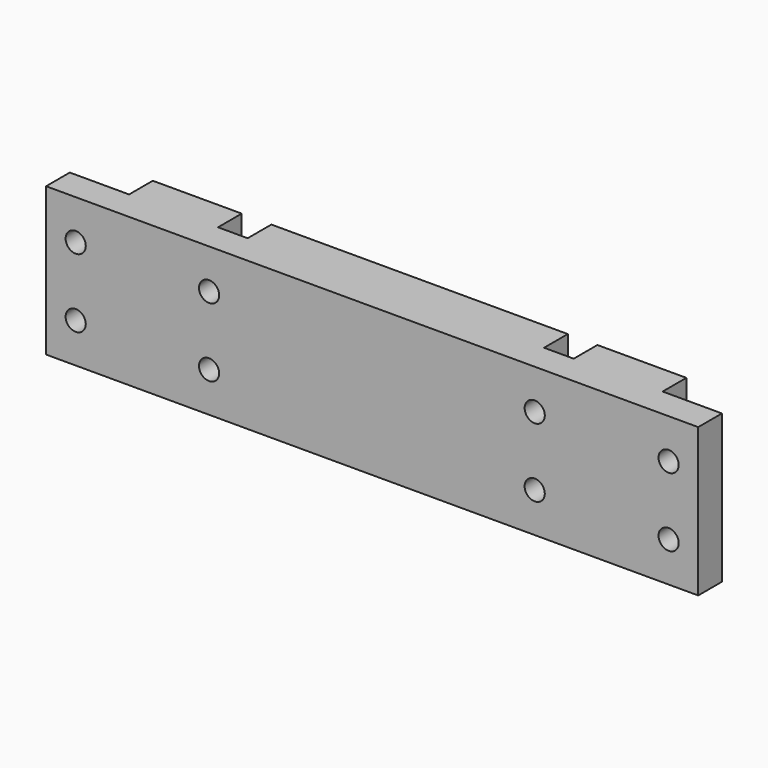
from build123d import *

# Parameters (mm, degrees)
F0_W      = 12.7
F0_H      = 31.75
F1_DEPTH  = 139.7
F2_W      = 12.7
F2_H      = 6.35
F2_W_2    = 6.35
F3_DEPTH  = 31.751
F4_R      = 2.159
F5_DEPTH  = 25.4
F6_R      = 2.159
F7_DEPTH  = 25.4
F8_W      = 50.8
F8_H      = 19.05
F9_DEPTH  = 6.35
F10_W     = 6.35
F10_H     = 19.05
F11_DEPTH = 6.35
F12_R     = 3.17499


# Not quite as in the source:
# - a fillet or chamfer is up to 0.001 mm smaller than in the source, because OpenCascade refuses the exact size


with BuildPart() as f1:
    # F0 (on Right) → F1 (new body)
    with BuildSketch(Plane.YZ):
        with Locations((6.35, 15.875)):
            Rectangle(F0_W, F0_H)
    extrude(amount=F1_DEPTH)

    # F2 (on face) → F3 (cut, through all)
    with BuildSketch(Plane.XY.offset(31.75)):
        with Locations((6.35, 9.525)):
            Rectangle(F2_W, F2_H)
        with Locations((34.925, 9.525)):
            Rectangle(F2_W_2, F2_H)
        with Locations((104.775, 9.525)):
            Rectangle(F2_W_2, F2_H)
        with Locations((133.35, 9.525)):
            Rectangle(F2_W, F2_H)
    extrude(amount=-F3_DEPTH, mode=Mode.SUBTRACT)

    # F4 (on face) → F5 (cut)
    with BuildSketch(Plane.XZ):
        with Locations((6.3445889391, 23.241)):
            Circle(F4_R)
        with Locations((6.3445889391, 8.509)):
            Circle(F4_R)
        with BuildLine():
            ThreePointArc((135.5180395808, 8.509), (133.3590395808, 10.668), (131.2000395808, 8.509))
            ThreePointArc((131.2000395808, 8.509), (133.3590395808, 6.35), (135.5180395808, 8.509))
        make_face()
        with BuildLine():
            ThreePointArc((135.5180395808, 23.241), (133.3590395808, 25.4), (131.2000395808, 23.241))
            ThreePointArc((131.2000395808, 23.241), (133.3590395808, 21.082), (135.5180395808, 23.241))
        make_face()
    extrude(amount=-F5_DEPTH, mode=Mode.SUBTRACT)

    # F6 (on face) → F7 (cut)
    with BuildSketch(Plane.XZ):
        with Locations((34.9172241986, 23.241)):
            Circle(F6_R)
        with Locations((34.9172241986, 8.509)):
            Circle(F6_R)
        with Locations((104.6765521169, 8.509)):
            Circle(F6_R)
        with Locations((104.6765521169, 23.241)):
            Circle(F6_R)
    extrude(amount=-F7_DEPTH, mode=Mode.SUBTRACT)

    # F8 (on face) → F9 (cut)
    with BuildSketch(Plane(origin=(0, 12.7, 0), x_dir=(-1, 0, 0), z_dir=(0, 1, 0))):
        with Locations((-69.85, 15.875)):
            Rectangle(F8_W, F8_H)
    extrude(amount=-F9_DEPTH, mode=Mode.SUBTRACT)

    # F10 (on face) → F11 (cut)
    with BuildSketch(Plane(origin=(0, 12.7, 0), x_dir=(-1, 0, 0), z_dir=(0, 1, 0))):
        with Locations((-22.225, 15.875)):
            Rectangle(F10_W, F10_H)
        with Locations((-117.475, 15.875)):
            Rectangle(F10_W, F10_H)
    extrude(amount=-F11_DEPTH, mode=Mode.SUBTRACT)

    # F12 (radius 3.175 in the source; OpenCascade refuses exactly that, so slightly less here)
    f12_edges = [f1.edges().sort_by_distance(p)[0] for p in [
        (19.05, 9.525, 6.35),
        (25.4, 9.525, 6.35),
        (19.05, 9.525, 25.4),
        (25.4, 9.525, 25.4),
        (44.45, 9.525, 6.35),
        (95.25, 9.525, 6.35),
        (95.25, 9.525, 25.4),
        (44.45, 9.525, 25.4),
        (120.65, 9.525, 6.35),
        (120.65, 9.525, 25.4),
        (114.3, 9.525, 25.4),
        (114.3, 9.525, 6.35),
    ]]
    fillet(f12_edges, radius=F12_R)


solid = f1.part
